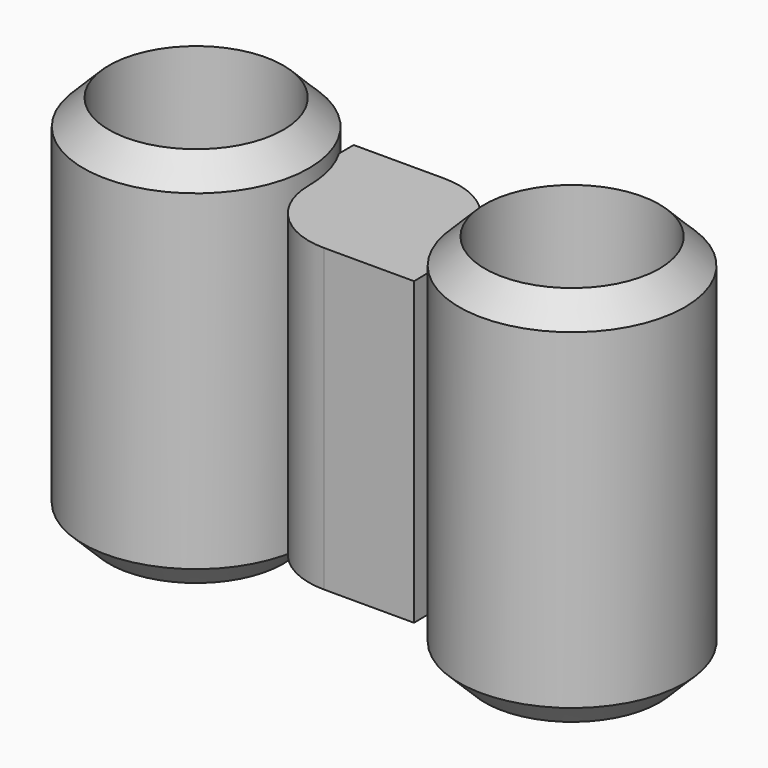
from build123d import *

# Parameters (mm, degrees)
F0_R     = 9.525
F0_R_2   = 7.366
F1_DEPTH = 19.05
F2_R     = 6.35
F3_DEPTH = 12.7
F4_W     = 7.6494621422
F4_H     = 6.35
F5_DEPTH = 12.7


# Not quite as in the source:
# - a fillet or chamfer that OpenCascade refuses, or shapes differently, is made with other operations: its cross-section is extruded or revolved along the edge and cut away or added


with BuildPart() as f1:
    # F0 (on Top) → F1 (new body, symmetric)
    with BuildSketch(Plane.XY):
        with Locations((-15.875, 0)):
            Circle(F0_R)
        with Locations((-15.875, 0)):
            Circle(F0_R_2, mode=Mode.SUBTRACT)
    extrude(amount=F1_DEPTH, both=True)



with BuildPart() as f1b:
    # F0 (on Top) → F1, piece 2 (new body, symmetric)
    with BuildSketch(Plane.XY):
        with Locations((15.875, 0)):
            Circle(F0_R)
        with Locations((15.875, 0)):
            Circle(F0_R_2, mode=Mode.SUBTRACT)
    extrude(amount=F1_DEPTH, both=True)


with BuildPart() as f1_1:
    add(f1.part)

    add(f1b.part)  # F3 merges F1b
    # F2 (on Top) → F3 (join, symmetric)
    with BuildSketch(Plane.XY):
        Circle(F2_R)
    extrude(amount=F3_DEPTH, both=True)

    # F4 (on Top) → F5 (join, symmetric)
    with BuildSketch(Plane.XY):
        with Locations((-3.8247310711, 3.175)):
            Rectangle(F4_W, F4_H)
        Polygon((7.4973143637, 0), (0, 0), (0, -6.35), (7.6071062533, -6.35), align=None)
    extrude(amount=F5_DEPTH, both=True)

    # F6: chamfer of 5.08 on 4 edges, made by hand

    # F6_s1 → F6_t2 (revolve, cut)
    with BuildSketch(Plane.XZ):
        Polygon((25.4, 13.97), (20.32, 19.05), (25.4, 19.05), align=None)
    revolve(axis=Axis((15.875, 0, 19.05), (0, 0, 1)), mode=Mode.SUBTRACT)

    # F6_s3 → F6_t4 (revolve, cut)
    with BuildSketch(Plane.XZ):
        Polygon((-6.35, 13.97), (-11.43, 19.05), (-6.35, 19.05), align=None)
    revolve(axis=Axis((-15.875, 0, 19.05), (0, 0, 1)), mode=Mode.SUBTRACT)

    # F6_s5 → F6_t6 (revolve, cut)
    with BuildSketch(Plane.XZ):
        Polygon((25.4, -13.97), (20.32, -19.05), (25.4, -19.05), align=None)
    revolve(axis=Axis((15.875, 0, -19.05), (0, 0, 1)), mode=Mode.SUBTRACT)

    # F6_s7 → F6_t8 (revolve, cut)
    with BuildSketch(Plane.XZ):
        Polygon((-6.35, -13.97), (-11.43, -19.05), (-6.35, -19.05), align=None)
    revolve(axis=Axis((-15.875, 0, -19.05), (0, 0, 1)), mode=Mode.SUBTRACT)


solid = f1_1.part
